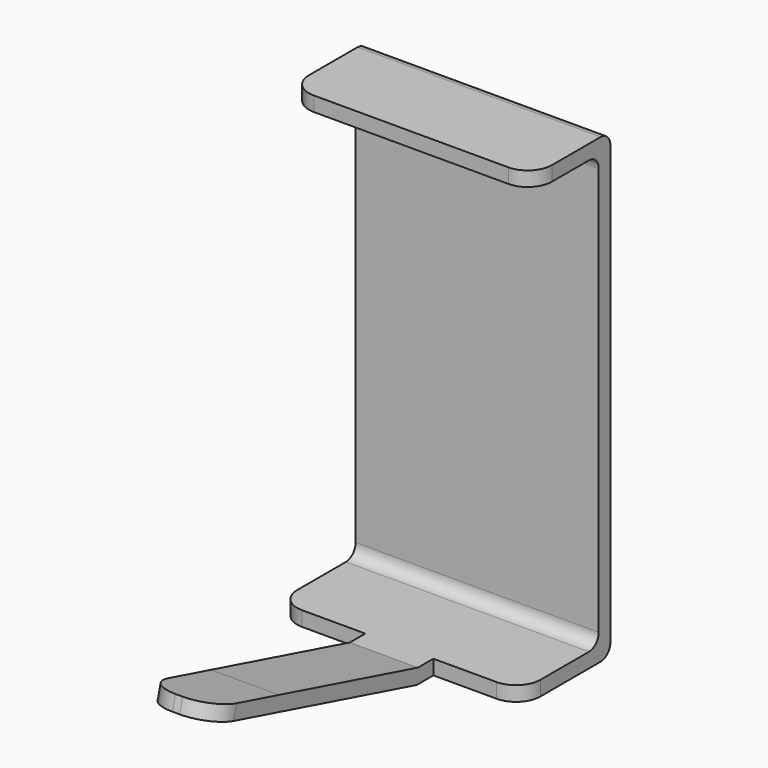
from build123d import *

# Parameters (mm, degrees)
F0_W     = 1.2
F0_H     = 1.2
F0_W_2   = 6.8
F0_H_2   = 35.5907311706
F0_H_3   = 1.2092688294
F1_DEPTH = 20
F3_DEPTH = 40.4
F4_R     = 2
F5_R     = 2.5
F6_R     = 2
F7_R     = 1


# Not quite as in the source:
# - ends of sketch curves that miss each other by under 0.0002 mm in the source are joined


with BuildPart() as f1:
    # F0 (on Right) → F1 (new body)
    with BuildSketch(Plane.YZ):
        with Locations((-0.6, 82.4221718073)):
            Rectangle(F0_W, F0_H)
        with Locations((-4.6, 82.4221718073)):
            Rectangle(F0_W_2, F0_H)
        with Locations((-0.6, 64.026806222)):
            Rectangle(F0_W, F0_H_2)
        with Locations((-0.6, 45.626806222)):
            Rectangle(F0_W, F0_H_3)
        Polygon((-1.2, 45.0221718073), (-1.2, 46.2314406367), (-10.7555877391, 46.2314406367), (-10.7812210649, 46.2314406367), (-10.8245881359, 46.2430607959), (-25.0829152046, 50.0635639224), (-31.8443964743, 51.8752954254), (-32.1549790177, 50.7161843506), (-25.393497748, 48.9044528476), (-10.9046093128, 45.0221710554), align=None)
    extrude(amount=F1_DEPTH)

    # F2 (on face) → F3 (cut)
    with BuildSketch(Plane.XY.offset(83.0221718073)):
        Polygon((7.2019821778, -9.2), (-6.1580585316, -9.2), (-6.1580585316, -39.2), (25.7106479257, -39.2), (25.7106479257, -9.2), (12.7980178222, -9.2), (12.7980178222, -35.1533853561), (7.2019821778, -35.1533853561), align=None)
    extrude(amount=-F3_DEPTH, mode=Mode.SUBTRACT)

    # F4
    f4_edges = [f1.edges().sort_by_distance(p)[0] for p in [
        (0, -9.2, 45.626806),
        (20, -9.2, 45.626806),
    ]]
    fillet(f4_edges, radius=F4_R)

    # F5
    f5_edges = [f1.edges().sort_by_distance(p)[0] for p in [
        (12.798018, -31.999688, 51.29574),
        (7.201982, -31.999688, 51.29574),
    ]]
    fillet(f5_edges, radius=F5_R)

    # F6
    f6_edges = [f1.edges().sort_by_distance(p)[0] for p in [
        (20, -8, 82.422172),
        (0, -8, 82.422172),
    ]]
    fillet(f6_edges, radius=F6_R)

    # F7
    f7_edges = [f1.edges().sort_by_distance(p)[0] for p in [
        (10, -1.2, 46.231441),
        (10, 0, 45.022172),
        (10, 0, 83.022172),
        (10, -1.2, 81.822172),
    ]]
    fillet(f7_edges, radius=F7_R)


solid = f1.part
